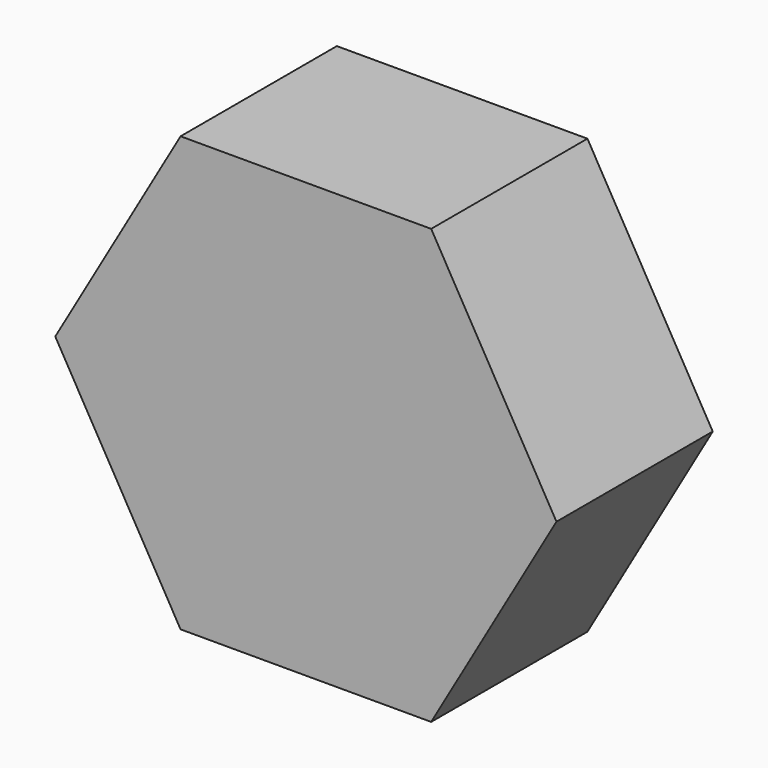
from build123d import *

# Parameters (mm, degrees)
F1_DEPTH = 7.14375


# Not quite as in the source:
# - a length typed as a fraction of an inch, garbled in the dataset ("3 / 203.2 mm" for 3/8 in), is restored


with BuildPart() as f1:
    # F0 (on Front) → F1 (new body)
    with BuildSketch(Plane.XZ):
        Polygon((4.5827177617, 7.9375), (-4.5827177617, 7.9375), (-9.1654355234, 0), (-4.5827177617, -7.9375), (4.5827177617, -7.9375), (9.1654355234, 0), align=None)
    extrude(amount=F1_DEPTH)


solid = f1.part
